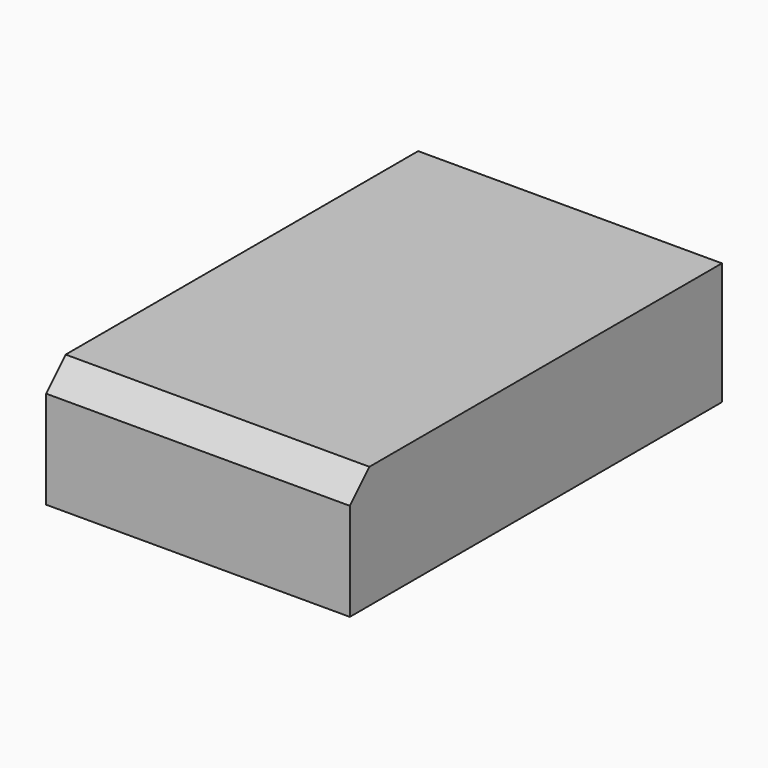
from build123d import *

# Parameters (mm, degrees)
F0_W     = 63.127156347
F0_H     = 96.6481640935
F1_DEPTH = 25.4
F2_SIZE  = 5.08


with BuildPart() as f1:
    # F0 (on Top) → F1 (new body)
    with BuildSketch(Plane.XY):
        with Locations((-31.5635781735, 0)):
            Rectangle(F0_W, F0_H)
    extrude(amount=F1_DEPTH)

    # F2
    f2_edges = [f1.edges().sort_by_distance(p)[0] for p in [
        (-31.563578, -48.324082, 25.4),
    ]]
    chamfer(f2_edges, length=F2_SIZE)


solid = f1.part
